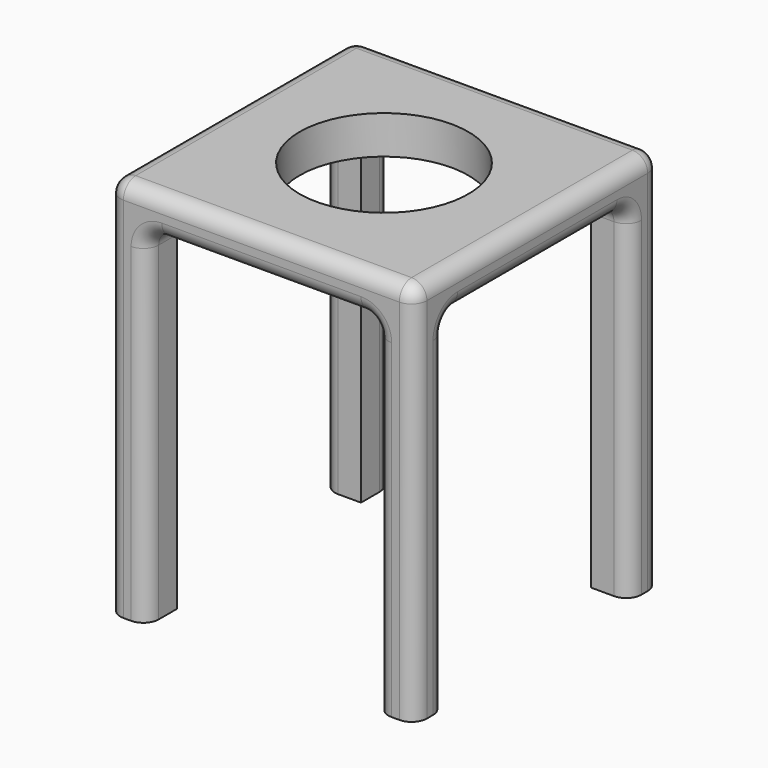
from build123d import *

# Parameters (mm, degrees)
F0_W     = 5
F0_H     = 5
F1_DEPTH = 50
F2_W     = 40
F2_H     = 40
F3_DEPTH = 5
F4_F1_R  = 2
F4_F2_R  = 2
F5_D     = 22
F5_DEPTH = 50
F5_START = 45
F5_TIP   = 6.6094668093


with BuildPart() as f1:
    # F0 (on Top) → F1 (new body)
    with BuildSketch(Plane.XY):
        with Locations((2.5, 2.5)):
            Rectangle(F0_W, F0_H)
    extrude(amount=F1_DEPTH)



with BuildPart() as f1b:
    # F0 (on Top) → F1, piece 2 (new body)
    with BuildSketch(Plane.XY):
        with Locations((37.5, 2.5)):
            Rectangle(F0_W, F0_H)
    extrude(amount=F1_DEPTH)


with BuildPart() as f1c:
    # F0 (on Top) → F1, piece 3 (new body)
    with BuildSketch(Plane.XY):
        with Locations((37.5, 37.5)):
            Rectangle(F0_W, F0_H)
    extrude(amount=F1_DEPTH)


with BuildPart() as f1d:
    # F0 (on Top) → F1, piece 4 (new body)
    with BuildSketch(Plane.XY):
        with Locations((2.5, 37.5)):
            Rectangle(F0_W, F0_H)
    extrude(amount=F1_DEPTH)


with BuildPart() as f1_1:
    add(f1.part)

    add(f1b.part)  # F3 merges F1b

    add(f1c.part)  # F3 merges F1c

    add(f1d.part)  # F3 merges F1d
    # F2 (on face) → F3 (join)
    with BuildSketch(Plane.XY.offset(50)):
        with Locations((20, 20)):
            Rectangle(F2_W, F2_H)
    extrude(amount=-F3_DEPTH)

    # F4: fillet of radius 2 on 20 edges, made by hand

    # F4_f1
    f4_f1_edges = [f1_1.edges().sort_by_distance(p)[0] for p in [
        (37.5, 5, 45),
        (35, 2.5, 45),
        (5, 2.5, 45),
        (2.5, 5, 45),
        (2.5, 35, 45),
        (5, 37.5, 45),
        (35, 37.5, 45),
        (37.5, 35, 45),
    ]]
    fillet(f4_f1_edges, radius=F4_F1_R)

    # F4_f2
    f4_f2_edges = [f1_1.edges().sort_by_distance(p)[0] for p in [
        (0, 20, 50),
        (20, 0, 50),
        (40, 20, 50),
        (20, 40, 50),
        (0, 0, 25),
        (40, 0, 25),
        (40, 40, 25),
        (20, 0, 45),
        (0, 20, 45),
        (20, 40, 45),
        (40, 20, 45),
        (0, 40, 25),
        (40, 5.5857864376, 44.4142135624),
        (40, 34.4142135624, 44.4142135624),
        (34.4142135624, 40, 44.4142135624),
        (5.5857864376, 40, 44.4142135624),
        (0, 34.4142135624, 44.4142135624),
        (0, 5.5857864376, 44.4142135624),
        (5.5857864376, 0, 44.4142135624),
        (34.4142135624, 0, 44.4142135624),
    ]]
    fillet(f4_f2_edges, radius=F4_F2_R)

    # F5
    # its depths count from where the whole tool has entered the part; down to there all is cleared
    with Locations(Plane(origin=(0, 0, 0), x_dir=(1, 0, 0), z_dir=(0, 0, -1)).offset(-F5_START)):
        with Locations((20, -20)):
            Hole(F5_D / 2, depth=F5_DEPTH)
            with Locations((0, 0, -(F5_DEPTH + F5_TIP / 2))):  # 118° drill point
                Cone(0, F5_D / 2, F5_TIP, mode=Mode.SUBTRACT)


solid = f1_1.part
